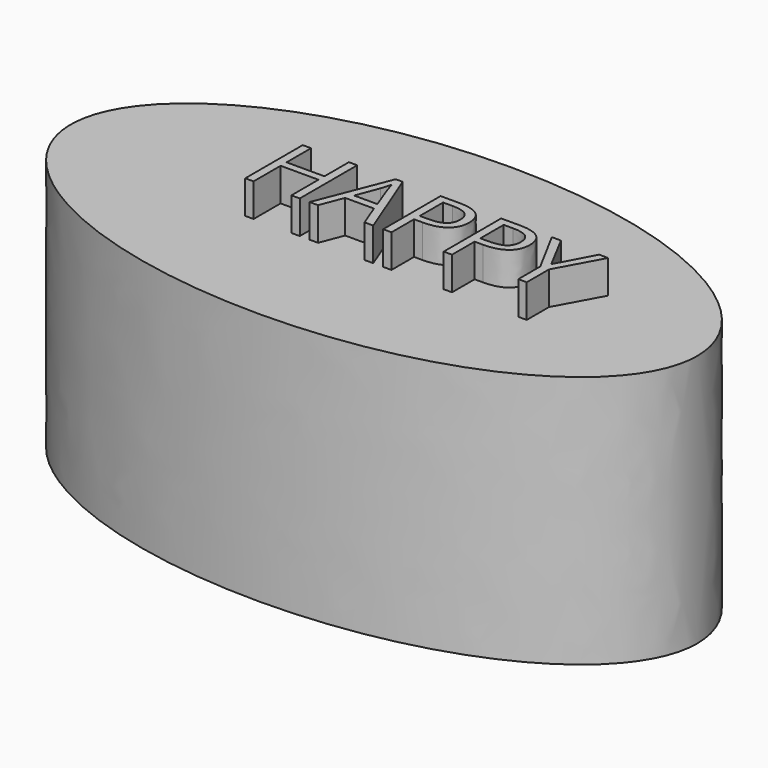
from build123d import *

# Parameters (mm, degrees)
F1_DEPTH     = 42.672
F2_TEXT_SIZE = 16.959208814
F3_DEPTH     = 5.588


# Not quite as in the source:
# - Text() gives the source's letters only with a copy of the font that has no kerning and outlines rounded to 1/6400 em; it was checked with that copy


with BuildPart() as f1:
    # F0 (on Top) → F1 (new body)
    with BuildSketch(Plane.XY):
        with BuildLine():
            add(Edge.make_bspline(
                [(35.2583751082, 0), (35.2583751082, 46.2414274517), (-43.9584972337, 23.1207137259), (-123.1753695756, 0), (-43.9584972337, -23.1207137259), (35.2583751082, -46.2414274517), (35.2583751082, 0)],
                knots=[0, 0, 0, 2.0943951024, 2.0943951024, 4.1887902048, 4.1887902048, 6.2831853072, 6.2831853072, 6.2831853072], degree=2, weights=[1, 0.5, 1, 0.5, 1, 0.5, 1]))
        make_face()
    extrude(amount=F1_DEPTH)

    # F2 (on face) → F3 (join)
    with BuildSketch(Plane.XY.offset(42.672)):
        with Locations((-37.8055982292, -6.0057034716)):
            Text('HAPPY', F2_TEXT_SIZE, font='Open Sans', text_align=(TextAlign.LEFT, TextAlign.BOTTOM))
    extrude(amount=F3_DEPTH)


solid = f1.part
